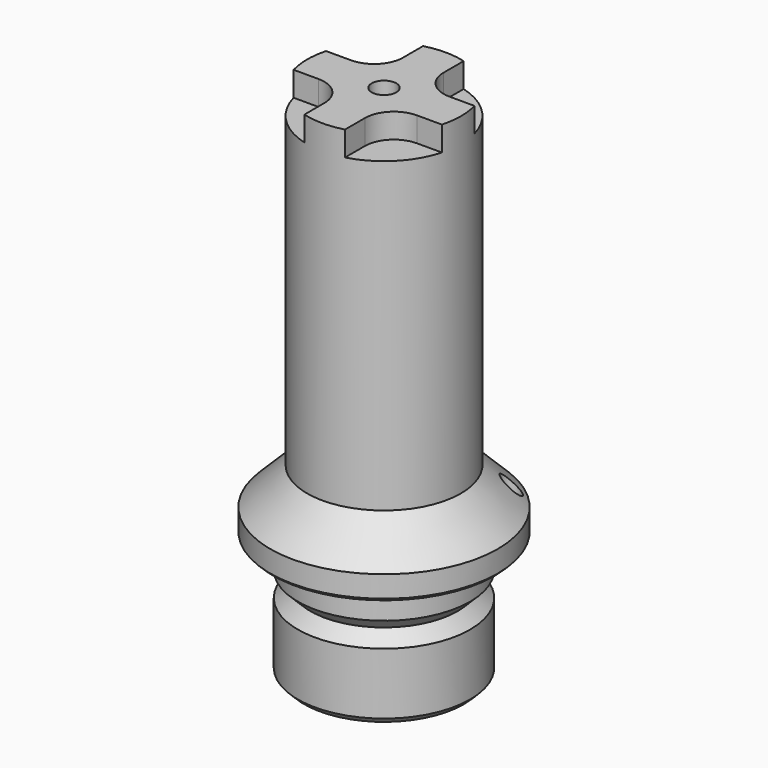
from build123d import *

# Parameters (mm, degrees)
F0_R         = 14
F1_DEPTH     = 80
F3_R         = 18.5
F4_DEPTH     = 4
F8_DEPTH     = 4
F9_R         = 4.7
F10_R        = 2
F11_DEPTH    = 84.001
F12_R        = 10
F12_R_2      = 2
F13_DEPTH    = 70
F14_SIZE     = 1
F15_SIZE     = 0.5
F16_R        = 1.5
F17_DEPTH    = 25
F18_R        = 14
F18_R_2      = 12.5
F19_DEPTH    = 60
F20_S5_R     = 1.5
F20_T6_DEPTH = 28
F20_S7_R     = 18.5
F20_T8_DEPTH = 28


# Not quite as in the source:
# - a fillet or chamfer that OpenCascade refuses, or shapes differently, is made with other operations: its cross-section is extruded or revolved along the edge and cut away or added


with BuildPart() as f1:
    # F0 (on Top) → F1 (new body)
    with BuildSketch(Plane.XY):
        Circle(F0_R)
    extrude(amount=F1_DEPTH)

    # F3 (on offset) → F4 (join)
    with BuildSketch(Plane(origin=(0, 0, 20), x_dir=(1, 0, 0), z_dir=(0, 0, -1))):
        Circle(F3_R)
    extrude(amount=-F4_DEPTH)

    # F5 (on Front) → F6 (revolve, cut)
    with BuildSketch(Plane.XZ):
        Polygon((14, 15), (12, 13), (14, 11), align=None)
    revolve(axis=Axis((0, 0, 15.3274592012), (0, 0, 1)), mode=Mode.SUBTRACT)

    # F7 (on face) → F8 (join)
    with BuildSketch(Plane.XY.offset(80)):
        with BuildLine():
            Line((-3.3, -3.3), (-3.3, 0))
            Line((-3.3, 0), (-3.3, 3.3))
            Line((-3.3, 3.3), (-13.6055135882, 3.3))
            ThreePointArc((-13.6055135882, 3.3), (-14, 0), (-13.6055135882, -3.3))
            Line((-13.6055135882, -3.3), (-3.3, -3.3))
        make_face()
        Polygon((-3.3, 3.3), (-3.3, 0), (-3.3, -3.3), (0, -3.3), (3.3, -3.3), (3.3, 0), (3.3, 3.3), (0, 3.3), align=None)
        with BuildLine():
            Line((-3.3, 13.6055135882), (-3.3, 3.3))
            Line((-3.3, 3.3), (0, 3.3))
            Line((0, 3.3), (3.3, 3.3))
            Line((3.3, 3.3), (3.3, 13.6055135882))
            ThreePointArc((3.3, 13.6055135882), (0, 14), (-3.3, 13.6055135882))
        make_face()
        with BuildLine():
            Line((0, -3.3), (-3.3, -3.3))
            Line((-3.3, -3.3), (-3.3, -13.6055135882))
            ThreePointArc((-3.3, -13.6055135882), (0, -14), (3.3, -13.6055135882))
            Line((3.3, -13.6055135882), (3.3, -3.3))
            Line((3.3, -3.3), (0, -3.3))
        make_face()
        with BuildLine():
            Line((13.6055135882, 3.3), (3.3, 3.3))
            Line((3.3, 3.3), (3.3, 0))
            Line((3.3, 0), (3.3, -3.3))
            Line((3.3, -3.3), (13.6055135882, -3.3))
            ThreePointArc((13.6055135882, -3.3), (14, 0), (13.6055135882, 3.3))
        make_face()
    extrude(amount=F8_DEPTH)

    # F9
    f9_edges = [f1.edges().sort_by_distance(p)[0] for p in [
        (-3.3, 3.3, 82),
        (3.3, 3.3, 82),
        (3.3, -3.3, 82),
        (-3.3, -3.3, 82),
    ]]
    fillet(f9_edges, radius=F9_R)

    # F10 (on face) → F11 (cut, through all)
    with BuildSketch(Plane.XY.offset(84)):
        Circle(F10_R)
    extrude(amount=-F11_DEPTH, mode=Mode.SUBTRACT)

    # F12 (on face) + F8_face1 (on face) → F13 (cut)
    with BuildSketch(Plane(origin=(0, 0, 0), x_dir=(1, 0, 0), z_dir=(0, 0, -1))):
        Circle(F12_R)
        Circle(F12_R_2, mode=Mode.SUBTRACT)
        Circle(F12_R)
    with BuildSketch(Plane(origin=(-7.5775327369, -7.5775327369, 80), x_dir=(1, 0, 0), z_dir=(0, 0, 1))):
        with BuildLine():
            Line((-0.4224672631, 4.2775327369), (-6.0279808513, 4.2775327369))
            ThreePointArc((-6.0279808513, 4.2775327369), (-2.3219621997, -2.3219621997), (4.2775327369, -6.0279808513))
            Line((4.2775327369, -6.0279808513), (4.2775327369, -0.4224672631))
            ThreePointArc((4.2775327369, -0.4224672631), (2.9009346085, 2.9009346085), (-0.4224672631, 4.2775327369))
        make_face()
    extrude(amount=-F13_DEPTH, dir=(0, 0, -1), mode=Mode.SUBTRACT)

    # F14
    f14_edges = [f1.edges().sort_by_distance(p)[0] for p in [
        (-14, 0, 0),
    ]]
    chamfer(f14_edges, length=F14_SIZE)

    # F15
    f15_edges = [f1.edges().sort_by_distance(p)[0] for p in [
        (-18.5, 0, 20),
    ]]
    chamfer(f15_edges, length=F15_SIZE)

    # F16 (on face) → F17 (cut)
    with BuildSketch(Plane(origin=(0, 0, 20), x_dir=(1, 0, 0), z_dir=(0, 0, -1))):
        with Locations((11.4904851943, -11.4904851943)):
            Circle(F16_R)
    extrude(amount=-F17_DEPTH, mode=Mode.SUBTRACT)

    # F18 (on face) → F19 (cut, through all)
    with BuildSketch(Plane.XY.offset(84)):
        Circle(F18_R)
        Circle(F18_R_2, mode=Mode.SUBTRACT)
    extrude(amount=-F19_DEPTH, mode=Mode.SUBTRACT)

    # F20: chamfer of 6 on 1 edges, made by hand


with BuildPart() as f20_tool2:
    # F20_s3 → F20_t4 (revolve)
    with BuildSketch(Plane.XZ):
        Polygon((18.5, 24), (12.5, 30), (12.5, 24), align=None)
    revolve(axis=Axis((0, 0, 24), (0, 0, 1)))

    # F20_s5 → F20_t6 (cut, symmetric)
    with BuildSketch(Plane.XY.offset(27)):
        with Locations((11.4904851943, 11.4904851943)):
            Circle(F20_S5_R)
    extrude(amount=F20_T6_DEPTH, both=True, mode=Mode.SUBTRACT)

    # F20_s7 → F20_t8 (intersect, symmetric)
    with BuildSketch(Plane.XY.offset(27)):
        Circle(F20_S7_R)
    extrude(amount=F20_T8_DEPTH, both=True, mode=Mode.INTERSECT)


with BuildPart() as f1_1:
    add(f1.part)

    # F20_t1: union F20_tool2
    add(f20_tool2.part)


solid = f1_1.part
